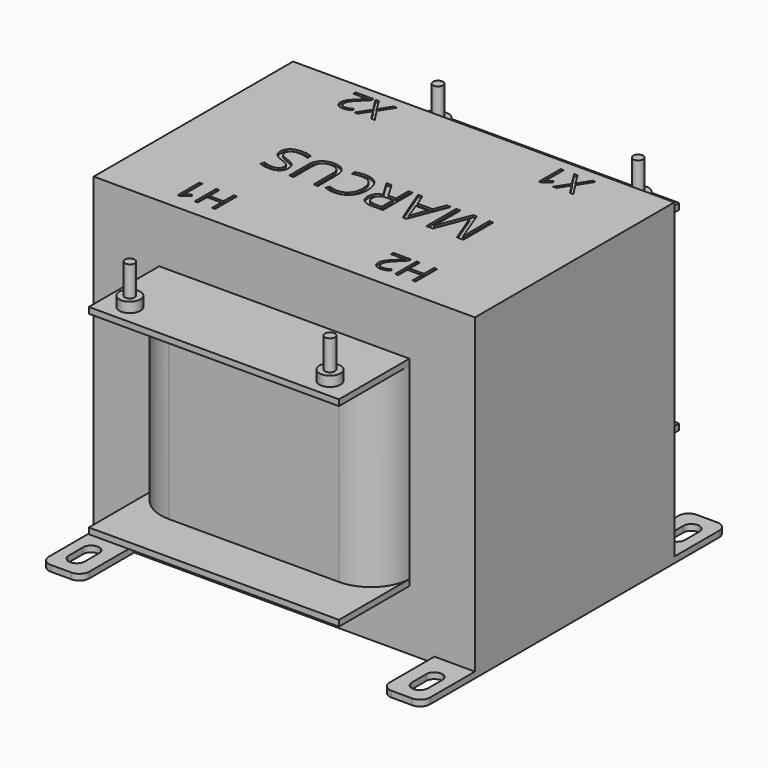
from build123d import *

# Parameters (mm, degrees)
F1_DEPTH        = 3
F2_W            = 190.5
F2_H            = 124.5
F3_DEPTH        = 155.8
F4_W            = 125
F4_H            = 100
F5_DEPTH        = 44
F6_W            = 125
F6_H            = 100
F7_DEPTH        = 44
F9_DEPTH        = 158.801
F10_R           = 5.25
F11_DEPTH       = 5
F12_R           = 2.5
F13_DEPTH       = 15
F14_R           = 2.5
F15_DEPTH       = 15
F16_R           = 5.25
F17_DEPTH       = 5
F18_R           = 2.5
F19_DEPTH       = 15
F20_R           = 2.5
F21_DEPTH       = 15
F22_W           = 25
F22_H           = 94
F23_DEPTH       = 157.751
F24_W           = 25
F24_H           = 94
F25_DEPTH       = 157.751
F26_T1_DEPTH    = 94
F27_T1_DEPTH    = 94
F28_R           = 5
F29_TEXT_SIZE   = 26.1712301936
F29_TEXT_SIZE_2 = 18.932375436
F30_DEPTH       = 1


# Not quite as in the source:
# - a fillet or chamfer that OpenCascade refuses, or shapes differently, is made with other operations: its cross-section is extruded or revolved along the edge and cut away or added
# - Text() gives the source's letters only with a copy of the font that has no kerning and outlines rounded to 1/6400 em; it was checked with that copy


with BuildPart() as f1:
    # F0 (on Top) → F1 (new body)
    with BuildSketch(Plane.XY):
        Polygon((0, 191.8134945184), (0, 1.3134945184), (20.25, 1.3134945184), (20.25, 34.3134945184), (170.25, 34.3134945184), (170.25, 1.3134945184), (190.5, 1.3134945184), (190.5, 191.8134945184), (170.25, 191.8134945184), (170.25, 158.8134945184), (20.25, 158.8134945184), (20.25, 191.8134945184), align=None)
    extrude(amount=F1_DEPTH)

    # F2 (on face) → F3 (join)
    with BuildSketch(Plane.XY.offset(3)):
        with Locations((95.25, 96.5634945184)):
            Rectangle(F2_W, F2_H)
    extrude(amount=F3_DEPTH)

    # F4 (on face) → F5 (join)
    with BuildSketch(Plane(origin=(0, 158.8134945184, 0), x_dir=(-1, 0, 0), z_dir=(0, 1, 0))):
        with Locations((-95.25, 80)):
            Rectangle(F4_W, F4_H)
    extrude(amount=F5_DEPTH)

    # F6 (on face) → F7 (join)
    with BuildSketch(Plane.XZ.offset(-34.3134945184)):
        with Locations((95.25, 80)):
            Rectangle(F6_W, F6_H)
    extrude(amount=F7_DEPTH)

    # F8 (on face) → F9 (cut, through all)
    with BuildSketch(Plane(origin=(0, 0, 0), x_dir=(1, 0, 0), z_dir=(0, 0, -1))):
        with BuildLine():
            Line((5.5, -172.3134945184), (5.5, -181.3134945184))
            ThreePointArc((5.5, -181.3134945184), (9.5, -185.3134945184), (13.5, -181.3134945184))
            Line((13.5, -181.3134945184), (13.5, -172.3134945184))
            ThreePointArc((13.5, -172.3134945184), (9.5, -168.3134945184), (5.5, -172.3134945184))
        make_face()
        with BuildLine():
            ThreePointArc((5.5, -20.8134945184), (9.5, -24.8134945184), (13.5, -20.8134945184))
            Line((13.5, -20.8134945184), (13.5, -11.8134945184))
            ThreePointArc((13.5, -11.8134945184), (9.5, -7.8134945184), (5.5, -11.8134945184))
            Line((5.5, -11.8134945184), (5.5, -20.8134945184))
        make_face()
        with BuildLine():
            Line((177, -11.8134945184), (177, -20.8134945184))
            ThreePointArc((177, -20.8134945184), (181, -24.8134945184), (185, -20.8134945184))
            Line((185, -20.8134945184), (185, -11.8134945184))
            ThreePointArc((185, -11.8134945184), (181, -7.8134945184), (177, -11.8134945184))
        make_face()
        with BuildLine():
            ThreePointArc((177, -181.3134945184), (181, -185.3134945184), (185, -181.3134945184))
            Line((185, -181.3134945184), (185, -172.3134945184))
            ThreePointArc((185, -172.3134945184), (181, -168.3134945184), (177, -172.3134945184))
            Line((177, -172.3134945184), (177, -181.3134945184))
        make_face()
    extrude(amount=-F9_DEPTH, mode=Mode.SUBTRACT)

    # F10 (on face) → F11 (join)
    with BuildSketch(Plane.XY.offset(130)):
        with Locations((145.25, 192.8134945184)):
            Circle(F10_R)
        with Locations((45.25, 192.8134945184)):
            Circle(F10_R)
    extrude(amount=F11_DEPTH)

    # F12 (on face) → F13 (join)
    with BuildSketch(Plane.XY.offset(135)):
        with Locations((145.25, 192.8134945184)):
            Circle(F12_R)
    extrude(amount=F13_DEPTH)

    # F14 (on face) → F15 (join)
    with BuildSketch(Plane.XY.offset(135)):
        with Locations((45.25, 192.8134945184)):
            Circle(F14_R)
    extrude(amount=F15_DEPTH)

    # F16 (on face) → F17 (join)
    with BuildSketch(Plane.XY.offset(130)):
        with Locations((45.25, 0.3134945184)):
            Circle(F16_R)
        with Locations((145.25, 0.3134945184)):
            Circle(F16_R)
    extrude(amount=F17_DEPTH)

    # F18 (on face) → F19 (join)
    with BuildSketch(Plane.XY.offset(135)):
        with Locations((45.25, 0.3134945184)):
            Circle(F18_R)
    extrude(amount=F19_DEPTH)

    # F20 (on face) → F21 (join)
    with BuildSketch(Plane.XY.offset(135)):
        with Locations((145.25, 0.3134945184)):
            Circle(F20_R)
    extrude(amount=F21_DEPTH)

    # F22 (on face) → F23 (cut, through all)
    with BuildSketch(Plane.YZ.offset(157.75)):
        with Locations((2.8134945184, 80)):
            Rectangle(F22_W, F22_H)
    extrude(amount=-F23_DEPTH, mode=Mode.SUBTRACT)

    # F24 (on face) → F25 (cut, through all)
    with BuildSketch(Plane.YZ.offset(157.75)):
        with Locations((190.3134945184, 80)):
            Rectangle(F24_W, F24_H)
    extrude(amount=-F25_DEPTH, mode=Mode.SUBTRACT)

    # F26: fillet of radius 20 on 1 edges, made by hand

    # F26_s2 → F26_t1 (cut)
    with BuildSketch(Plane.XY.offset(33)):
        with BuildLine():
            ThreePointArc((32.75, 158.8134945184), (38.9409356033, 172.3048712646), (52.7249843554, 177.8134945184))
            Line((52.7249843554, 177.8134945184), (32.75, 177.8134945184))
            Line((32.75, 177.8134945184), (32.75, 158.8134945184))
        make_face()
    extrude(amount=F26_T1_DEPTH, mode=Mode.SUBTRACT)

    # F27: fillet of radius 20 on 3 edges, made by hand

    # F27_s2 → F27_t1 (cut)
    with BuildSketch(Plane.XY.offset(33)):
        with BuildLine():
            ThreePointArc((137.7750156446, 177.8134945184), (151.5590643967, 172.3048712646), (157.75, 158.8134945184))
            Line((157.75, 158.8134945184), (157.75, 177.8134945184))
            Line((157.75, 177.8134945184), (137.7750156446, 177.8134945184))
        make_face()
        with BuildLine():
            ThreePointArc((52.7249843554, 15.3134945184), (38.9409356033, 20.8221177722), (32.75, 34.3134945184))
            Line((32.75, 34.3134945184), (32.75, 15.3134945184))
            Line((32.75, 15.3134945184), (52.7249843554, 15.3134945184))
        make_face()
        with BuildLine():
            ThreePointArc((137.7750156446, 15.3134945184), (151.5590643967, 20.8221177722), (157.75, 34.3134945184))
            Line((157.75, 34.3134945184), (157.75, 15.3134945184))
            Line((157.75, 15.3134945184), (137.7750156446, 15.3134945184))
        make_face()
    extrude(amount=F27_T1_DEPTH, mode=Mode.SUBTRACT)

    # F28
    f28_edges = [f1.edges().sort_by_distance(p)[0] for p in [
        (0, 1.313495, 1.5),
        (20.25, 1.313495, 1.5),
        (170.25, 1.313495, 1.5),
        (190.5, 1.313495, 1.5),
        (190.5, 191.813495, 1.5),
        (170.25, 191.813495, 1.5),
        (20.25, 191.813495, 1.5),
        (0, 191.813495, 1.5),
    ]]
    fillet(f28_edges, radius=F28_R)

    # F29 (on face) → F30 (cut)
    with BuildSketch(Plane.XY.offset(158.8)):
        with Locations(Location((148.5724970698, 101.3745516539), (0, 0, 180))):
            Text('MARCUS', F29_TEXT_SIZE, font='Open Sans', text_align=(TextAlign.LEFT, TextAlign.BOTTOM))
        with Locations(Location((55.9616908431, 56.070484221), (0, 0, -180))):
            Text('H1', F29_TEXT_SIZE_2, font='Open Sans', text_align=(TextAlign.LEFT, TextAlign.BOTTOM))
        with Locations(Location((155.3503200412, 56.9964945317), (0, 0, 180))):
            Text('H2', F29_TEXT_SIZE_2, font='Open Sans', text_align=(TextAlign.LEFT, TextAlign.BOTTOM))
        with Locations(Location((155.843757093, 153.1034260988), (0, 0, -180))):
            Text('X1', F29_TEXT_SIZE_2, font='Open Sans', text_align=(TextAlign.LEFT, TextAlign.BOTTOM))
        with Locations(Location((56.1242327095, 153.6759063601), (0, 0, 180))):
            Text('X2', F29_TEXT_SIZE_2, font='Open Sans', text_align=(TextAlign.LEFT, TextAlign.BOTTOM))
    extrude(amount=-F30_DEPTH, mode=Mode.SUBTRACT)


solid = f1.part
